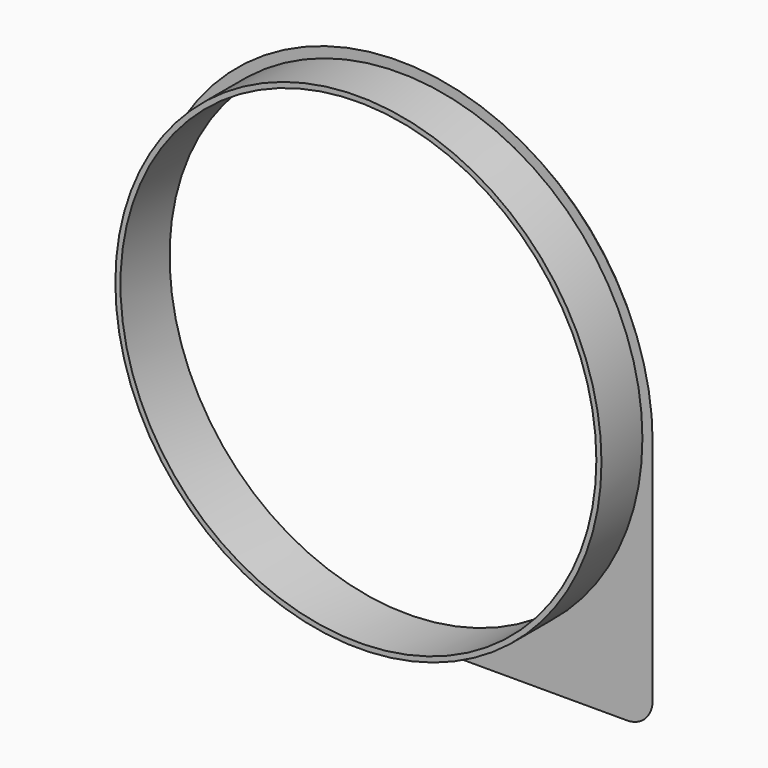
from build123d import *

# Parameters (mm, degrees)
F0_R     = 47.5
F0_R_2   = 46.5
F1_DEPTH = 2
F2_DEPTH = 12
F3_SIZE  = 1.99999


# Not quite as in the source:
# - a fillet or chamfer is up to 0.001 mm smaller than in the source, because OpenCascade refuses the exact size


with BuildPart() as f1:
    # F0 (on Front) → F1 (new body)
    with BuildSketch(Plane.XZ):
        with BuildLine():
            ThreePointArc((0, -49.5), (35.0017856687, -35.0017856687), (49.5, 0))
            ThreePointArc((49.5, 0), (-35.0017856687, 35.0017856687), (0, -49.5))
        make_face()
        Circle(F0_R, mode=Mode.SUBTRACT)
        Circle(F0_R)
        Circle(F0_R_2, mode=Mode.SUBTRACT)
        with BuildLine():
            Line((49.5, -44.5), (49.5, 0))
            ThreePointArc((49.5, 0), (35.0017856687, -35.0017856687), (0, -49.5))
            Line((0, -49.5), (44.5, -49.5))
            ThreePointArc((44.5, -49.5), (48.0355339059, -48.0355339059), (49.5, -44.5))
        make_face()
    extrude(amount=F1_DEPTH)

    # F0 (on Front) → F2 (join)
    with BuildSketch(Plane.XZ):
        Circle(F0_R)
        Circle(F0_R_2, mode=Mode.SUBTRACT)
    extrude(amount=F2_DEPTH)

    # F3 (size 2 in the source; OpenCascade refuses exactly that, so slightly less here)
    f3_edges = [f1.edges().sort_by_distance(p)[0] for p in [
        (49.5, 0, -22.25),
    ]]
    chamfer(f3_edges, length=F3_SIZE)


solid = f1.part
